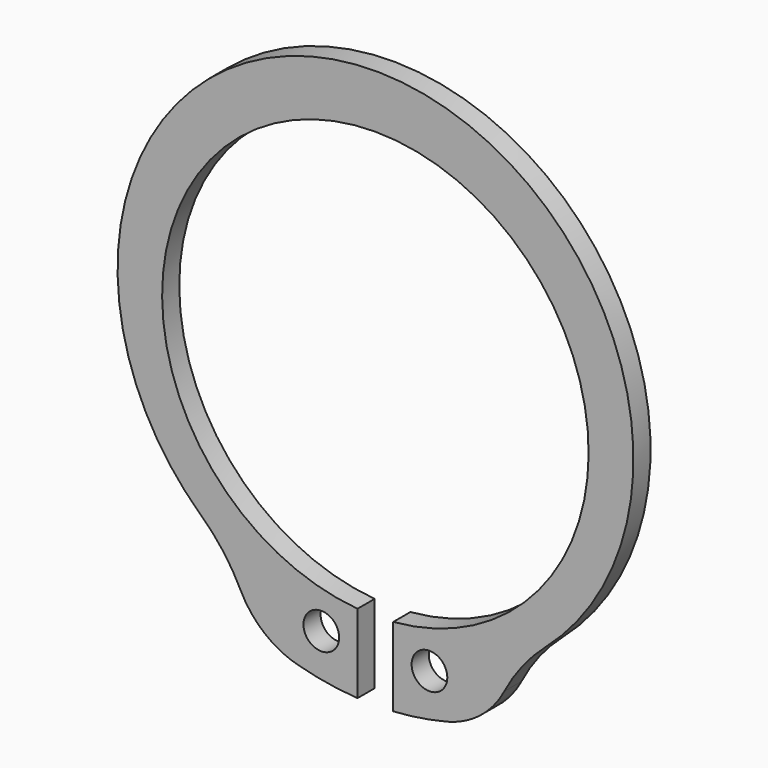
from build123d import *

# Parameters (mm, degrees)
F0_R        = 1
F1_DEPTH    = 1.2
F2_T1_DEPTH = 1.2
F3_R        = 5


# Not quite as in the source:
# - a fillet or chamfer that OpenCascade refuses, or shapes differently, is made with other operations: its cross-section is extruded or revolved along the edge and cut away or added


with BuildPart() as f1:
    # F0 (on Front) → F1 (new body)
    with BuildSketch(Plane.XZ):
        with BuildLine():
            ThreePointArc((-1, -11.9080854884), (0, 11.95), (1, -11.9080854884))
            Line((1, -11.9080854884), (1, -16.3193903072))
            ThreePointArc((1, -16.3193903072), (3.8276067146, -15.8956574837), (6.5381625357, -14.9858243236))
            Line((6.5381625357, -14.9858243236), (5.5446488339, -12.8552273145))
            ThreePointArc((5.5446488339, -12.8552273145), (0.2154334831, 14.9485032399), (-5.9128007498, -12.6901058819))
            Line((-5.9128007498, -12.6901058819), (-6.90530659, -14.8202307977))
            ThreePointArc((-6.90530659, -14.8202307977), (-4.0231005306, -15.8473077247), (-1, -16.3193903072))
            Line((-1, -16.3193903072), (-1, -11.9080854884))
        make_face()
        with Locations((-3.0301545951, -13.6681440997)):
            Circle(F0_R, mode=Mode.SUBTRACT)
        with Locations((3.0301545951, -13.6681440997)):
            Circle(F0_R, mode=Mode.SUBTRACT)
    extrude(amount=F1_DEPTH)

    # F2: fillet of radius 10 on 2 edges, made by hand

    # F2_s2 → F2_t1 (join)
    with BuildSketch(Plane.XZ):
        with BuildLine():
            ThreePointArc((-9.7709471746, -10.1486206785), (-8.0118480734, -12.2842810829), (-6.90530659, -14.8202307977))
            Line((-6.90530659, -14.8202307977), (-5.9128007498, -12.6901058819))
            ThreePointArc((-5.9128007498, -12.6901058819), (-7.9440740778, -11.5745099677), (-9.7709471746, -10.1486206785))
        make_face()
        with BuildLine():
            ThreePointArc((6.5381625357, -14.9858243236), (7.7071981674, -12.4786621044), (9.5183975603, -10.3877141232))
            ThreePointArc((9.5183975603, -10.3877141232), (7.6320006174, -11.7832822229), (5.5446488339, -12.8552273145))
            Line((5.5446488339, -12.8552273145), (6.5381625357, -14.9858243236))
        make_face()
    extrude(amount=F2_T1_DEPTH)

    # F3
    f3_edges = [f1.edges().sort_by_distance(p)[0] for p in [
        (-6.905307, -0.6, -14.820231),
        (6.538163, -0.6, -14.985824),
    ]]
    fillet(f3_edges, radius=F3_R)


solid = f1.part
